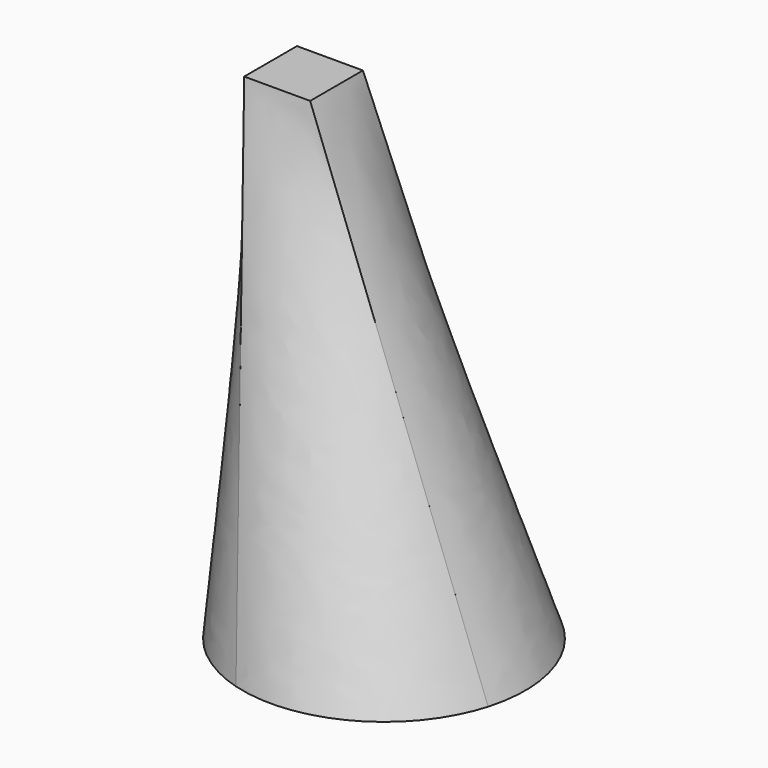
from build123d import *

# Parameters (mm, degrees)
F0_W = 7
F0_H = 7


# Not quite as in the source:
# - the arcs of a loft's sections are written as splines that run evenly, so that the points pair up as in the source's solid


with BuildPart() as f3:
    # F0 (on Top) → F3 section 0
    with BuildSketch(Plane.XY):
        with Locations((3.5, 0)):
            Rectangle(F0_W, F0_H)
    # F2 (on offset) → F3 section 1
    with BuildSketch(Plane.XY.offset(-50)):
        with BuildLine():
            add(Edge.make_bspline(
                [(-2.3670398878, 4.1883006664), (-2.915287163, 2.3028990793), (-3.0884365913, 0.3092290616), (-2.6584415625, -3.5941491101), (-2.05546629, -5.5023214516), (-0.1644445272, -8.9440206786), (1.1228579268, -10.4761934025), (4.1870155024, -12.9322461765), (5.9626650088, -13.8551598748), (7.8480665958, -14.40340715)],
                knots=[0, 0, 0, 0, 0.25, 0.25, 0.5, 0.5, 0.75, 0.75, 1, 1, 1, 1], degree=3))
            add(Edge.make_bspline(
                [(7.8480665958, -14.40340715), (9.7334681829, -14.9516544252), (11.7271382006, -15.1248038535), (15.6305163723, -14.6948088247), (17.5386887138, -14.0918335522), (20.9803879408, -12.2008117894), (22.5125606647, -10.9135093353), (24.9686134387, -7.8493517598), (25.891527137, -6.0737022534), (26.4397744122, -4.1883006664)],
                knots=[0, 0, 0, 0, 0.25, 0.25, 0.5, 0.5, 0.75, 0.75, 1, 1, 1, 1], degree=3))
            add(Edge.make_bspline(
                [(26.4397744122, -4.1883006664), (26.9880216874, -2.3028990793), (27.1611711157, -0.3092290616), (26.7311760869, 3.5941491101), (26.1282008144, 5.5023214516), (24.2371790516, 8.9440206786), (22.9498765975, 10.4761934025), (19.885719022, 12.9322461765), (18.1100695156, 13.8551598748), (16.2246679286, 14.40340715)],
                knots=[0, 0, 0, 0, 0.25, 0.25, 0.5, 0.5, 0.75, 0.75, 1, 1, 1, 1], degree=3))
            add(Edge.make_bspline(
                [(16.2246679286, 14.40340715), (14.3392663415, 14.9516544252), (12.3455963238, 15.1248038535), (8.4422181521, 14.6948088247), (6.5340458106, 14.0918335522), (3.0923465836, 12.2008117894), (1.5601738597, 10.9135093353), (-0.8958789143, 7.8493517598), (-1.8187926126, 6.0737022534), (-2.3670398878, 4.1883006664)],
                knots=[0, 0, 0, 0, 0.25, 0.25, 0.5, 0.5, 0.75, 0.75, 1, 1, 1, 1], degree=3))
        make_face()
    loft(ruled=True)


solid = f3.part
